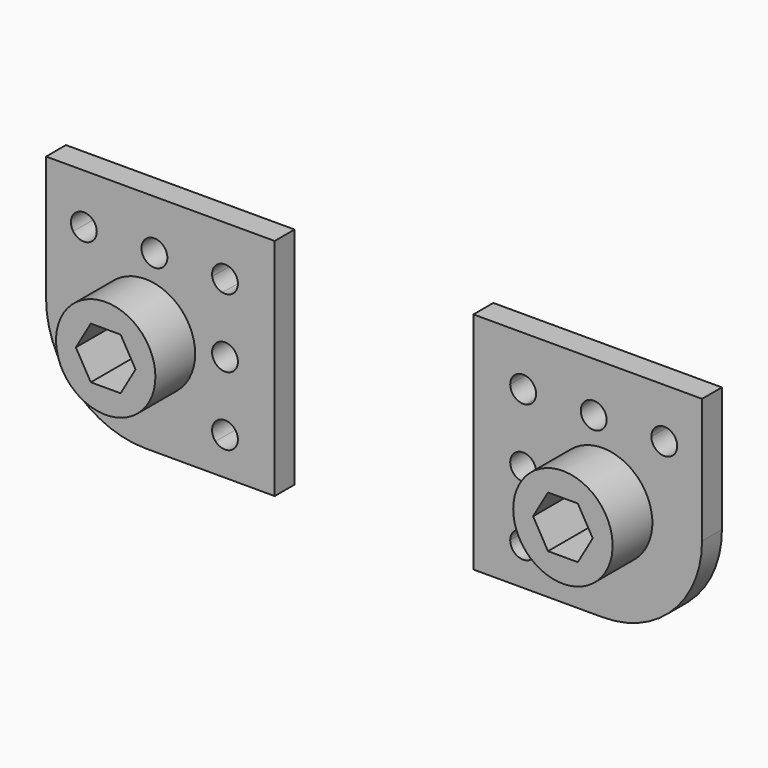
from build123d import *

# Parameters (mm, degrees)
F0_R     = 12.7
F0_R_2   = 3.302
F1_DEPTH = 6.35
F2_DEPTH = 19.05


# Not quite as in the source:
# - a feature names something its author has since deleted; it is built from what else it names


with BuildPart() as f1:
    # F0 (on Front) → F1 (new body)
    with BuildSketch(Plane.XZ):
        with BuildLine():
            Line((0, 0), (0, 25.4))
            Line((0, 25.4), (-58.4256423555, 25.4))
            Line((-58.4256423555, 25.4), (-58.4256423555, -6.604))
            ThreePointArc((-58.4256423555, -6.604), (-56.6297902297, 2.7770555445), (-51.4961775421, 10.8315765583))
            ThreePointArc((-51.4961775421, 10.8315765583), (-50.8609248096, 15.2586042986), (-46.3965154848, 14.9918271839))
            ThreePointArc((-46.3965154848, 14.9918271839), (-30.7169390659, 18.6908589465), (-15.9660970274, 12.2143929495))
            ThreePointArc((-15.9660970274, 12.2143929495), (-12.9434662353, 15.9930120243), (-9.398, 12.7))
            ThreePointArc((-9.398, 12.7), (-10.6088068714, 10.1445909723), (-13.3532485155, 9.4632623867))
            ThreePointArc((-13.3532485155, 9.4632623867), (-9.1003544415, 1.9248098954), (-7.6256423555, -6.604))
            ThreePointArc((-7.6256423555, -6.604), (-8.5138201304, -13.2621206963), (-11.1162385134, -19.4546040047))
            ThreePointArc((-11.1162385134, -19.4546040047), (-9.8598605291, -20.6677162396), (-9.398, -22.352))
            ThreePointArc((-9.398, -22.352), (-11.4864427084, -25.4229090999), (-15.1099822531, -24.609252653))
            ThreePointArc((-15.1099822531, -24.609252653), (-23.3347553317, -30.0826436724), (-33.0256423555, -32.004))
            Line((-33.0256423555, -32.004), (0, -32.004))
            Line((0, -32.004), (0, 0))
        make_face()
        with BuildLine():
            ThreePointArc((-51.4961775421, 10.8315765583), (-56.6297902297, 2.7770555445), (-58.4256423555, -6.604))
            ThreePointArc((-58.4256423555, -6.604), (-50.9861545976, -24.5645122421), (-33.0256423555, -32.004))
            ThreePointArc((-33.0256423555, -32.004), (-23.3347553317, -30.0826436724), (-15.1099822531, -24.609252653))
            ThreePointArc((-15.1099822531, -24.609252653), (-15.3102223776, -20.3296392163), (-11.1162385134, -19.4546040047))
            ThreePointArc((-11.1162385134, -19.4546040047), (-8.5138201304, -13.2621206963), (-7.6256423555, -6.604))
            ThreePointArc((-7.6256423555, -6.604), (-9.1003544415, 1.9248098954), (-13.3532485155, 9.4632623867))
            ThreePointArc((-13.3532485155, 9.4632623867), (-15.094263397, 10.4260811832), (-15.9660970274, 12.2143929495))
            ThreePointArc((-15.9660970274, 12.2143929495), (-30.7169390659, 18.6908589465), (-46.3965154848, 14.9918271839))
            ThreePointArc((-46.3965154848, 14.9918271839), (-45.7115779434, 13.9357044698), (-45.4716423555, 12.7))
            ThreePointArc((-45.4716423555, 12.7), (-47.795533769, 9.5461915732), (-51.4961775421, 10.8315765583))
        make_face()
        with Locations((-33.0256423555, -6.604)):
            Circle(F0_R, mode=Mode.SUBTRACT)
        with Locations((-12.7, -4.826)):
            Circle(F0_R_2, mode=Mode.SUBTRACT)
        with Locations((-30.7368211777, 12.7)):
            Circle(F0_R_2, mode=Mode.SUBTRACT)
    extrude(amount=F1_DEPTH)

    # F0 (on Front) → F2 (join)
    with BuildSketch(Plane.XZ):
        with Locations((-33.0256423555, -6.604)):
            Circle(F0_R)
        Polygon((-40.6512847109, -6.604), (-36.8384635332, 0), (-29.2128211777, 0), (-25.4, -6.604), (-29.2128211777, -13.208), (-36.8384635332, -13.208), align=None, mode=Mode.SUBTRACT)
    extrude(amount=F2_DEPTH)


with BuildPart() as f4_1:
    # F4: instance of F1
    add(f1.part.mirror(Plane.YZ.offset(25.4)))


solid = Compound([f1.part, f4_1.part])
